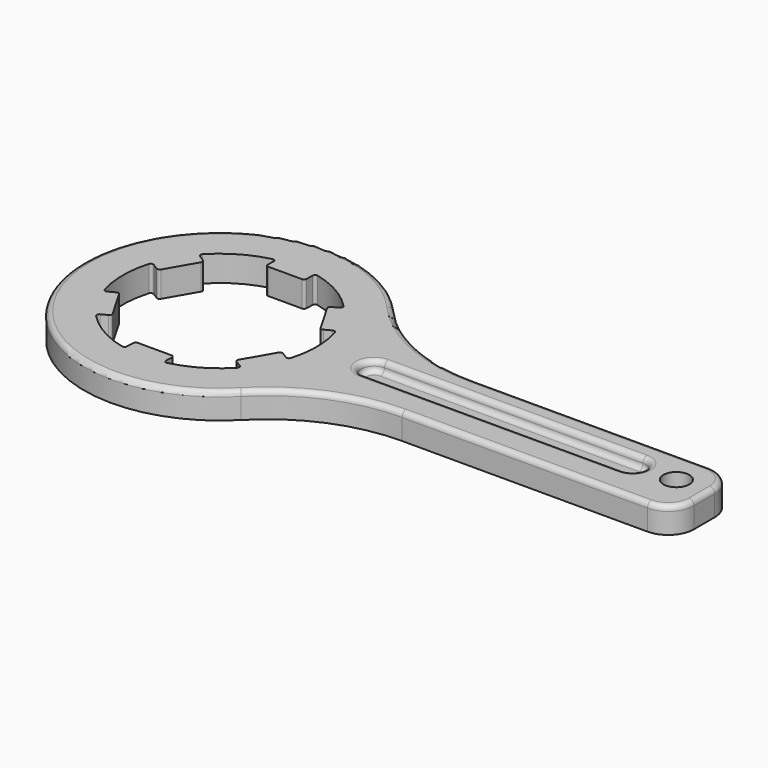
from build123d import *

# Parameters (mm, degrees)
F0_R     = 5
F1_DEPTH = 10
F2_R     = 10
F3_R     = 1
F4_DEPTH = 6
F5_R     = 1.99999
F6_R     = 2


# Not quite as in the source:
# - a fillet or chamfer is up to 0.001 mm smaller than in the source, because OpenCascade refuses the exact size


with BuildPart() as f1:
    # F0 (on Top) → F1 (new body)
    with BuildSketch(Plane.XY):
        with BuildLine():
            ThreePointArc((87.8922518749, 12.982062427), (61.2373823548, 18.6986926605), (39.2710061569, 34.8430491695))
            ThreePointArc((39.2710061569, 34.8430491695), (-52.4855584858, 1.231320604), (37.5938529252, -36.6463125326))
            ThreePointArc((37.5938529252, -36.6463125326), (58.881501719, -22.1257192654), (84.1386232135, -17.017937573))
            Line((84.1386232135, -17.017937573), (188.9996444946, -17.017937573))
            Line((188.9996444946, -17.017937573), (188.9996444946, 12.982062427))
            Line((188.9996444946, 12.982062427), (87.8922518749, 12.982062427))
        make_face()
        with BuildLine():
            ThreePointArc((-28.0871828778, 24.8467333464), (-18.7727000217, 32.4628361961), (-7.5256854941, 36.7370937588))
            Line((-7.5256854941, 36.7370937588), (-7.6951050263, 31.7399648809))
            Line((-7.6951050263, 31.7399648809), (7.3048913079, 31.7504516883))
            Line((7.3048913079, 31.7504516883), (7.4743108401, 36.7475805661))
            ThreePointArc((7.4743108401, 36.7475805661), (18.7272908139, 32.4890532145), (28.0524137093, 24.8859816982))
            Line((28.0524137093, 24.8859816982), (23.6400633889, 22.5341388781))
            Line((23.6400633889, 22.5341388781), (31.1491433976, 9.5490043996))
            Line((31.1491433976, 9.5490043996), (35.561493718, 11.9008472197))
            ThreePointArc((35.561493718, 11.9008472197), (37.4999908356, 0.0262170183), (35.5780992034, -11.8511120606))
            Line((35.5780992034, -11.8511120606), (31.3351684153, -9.2058260029))
            Line((31.3351684153, -9.2058260029), (23.8442520897, -22.2014472886))
            Line((23.8442520897, -22.2014472886), (28.0871828778, -24.8467333464))
            ThreePointArc((28.0871828778, -24.8467333464), (18.7727000217, -32.4628361961), (7.5256854941, -36.7370937588))
            Line((7.5256854941, -36.7370937588), (7.6951050263, -31.7399648809))
            Line((7.6951050263, -31.7399648809), (-7.3048913079, -31.7504516883))
            Line((-7.3048913079, -31.7504516883), (-7.4743108401, -36.7475805661))
            ThreePointArc((-7.4743108401, -36.7475805661), (-18.7272908139, -32.4890532145), (-28.0524137093, -24.8859816982))
            Line((-28.0524137093, -24.8859816982), (-23.6400633889, -22.5341388781))
            Line((-23.6400633889, -22.5341388781), (-31.1491433976, -9.5490043996))
            Line((-31.1491433976, -9.5490043996), (-35.561493718, -11.9008472197))
            ThreePointArc((-35.561493718, -11.9008472197), (-37.4999908356, -0.0262170183), (-35.5780992034, 11.8511120606))
            Line((-35.5780992034, 11.8511120606), (-31.3351684153, 9.2058260029))
            Line((-31.3351684153, 9.2058260029), (-23.8442520897, 22.2014472886))
            Line((-23.8442520897, 22.2014472886), (-28.0871828778, 24.8467333464))
        make_face(mode=Mode.SUBTRACT)
        with BuildLine():
            Line((159.6448034048, -5), (59.6448034048, -5))
            ThreePointArc((59.6448034048, -5), (54.6448034048, 0), (59.6448034048, 5))
            Line((59.6448034048, 5), (159.6448034048, 5))
            ThreePointArc((159.6448034048, 5), (164.6448034048, 0), (159.6448034048, -5))
        make_face(mode=Mode.SUBTRACT)
        with Locations((176.5601634979, 0)):
            Circle(F0_R, mode=Mode.SUBTRACT)
    extrude(amount=F1_DEPTH)

    # F2
    f2_edges = [f1.edges().sort_by_distance(p)[0] for p in [
        (188.999644, 12.982062, 5),
        (188.999644, -17.017938, 5),
    ]]
    fillet(f2_edges, radius=F2_R)

    # F3
    f3_edges = [f1.edges().sort_by_distance(p)[0] for p in [
        (-7.525685, 36.737094, 5),
        (-7.695105, 31.739965, 5),
        (7.304891, 31.750452, 5),
        (7.474311, 36.747581, 5),
        (23.640063, 22.534139, 5),
        (28.052414, 24.885982, 5),
        (31.149143, 9.549004, 5),
        (35.561494, 11.900847, 5),
        (35.578099, -11.851112, 5),
        (31.335168, -9.205826, 5),
        (23.844252, -22.201447, 5),
        (28.087183, -24.846733, 5),
        (7.525685, -36.737094, 5),
        (7.695105, -31.739965, 5),
        (-7.304891, -31.750452, 5),
        (-7.474311, -36.747581, 5),
        (-28.052414, -24.885982, 5),
        (-23.640063, -22.534139, 5),
        (-31.149143, -9.549004, 5),
        (-35.561494, -11.900847, 5),
        (-35.578099, 11.851112, 5),
        (-31.335168, 9.205826, 5),
        (-23.844252, 22.201447, 5),
        (-28.087183, 24.846733, 5),
    ]]
    fillet(f3_edges, radius=F3_R)

    # F0 (on Top) → F4 (join)
    with BuildSketch(Plane.XY):
        with BuildLine():
            ThreePointArc((59.6448034048, 5), (54.6448034048, 0), (59.6448034048, -5))
            Line((59.6448034048, -5), (159.6448034048, -5))
            ThreePointArc((159.6448034048, -5), (164.6448034048, 0), (159.6448034048, 5))
            Line((159.6448034048, 5), (59.6448034048, 5))
        make_face()
    extrude(amount=F4_DEPTH)

    # F5 (radius 2 in the source; OpenCascade refuses exactly that, so slightly less here)
    f5_edges = [f1.edges().sort_by_distance(p)[0] for p in [
        (109.644803, 5, 6),
        (109.644803, 5, 10),
    ]]
    fillet(f5_edges, radius=F5_R)

    # F6
    f6_edges = [f1.edges().sort_by_distance(p)[0] for p in [
        (-52.485558, 1.231321, 10),
    ]]
    fillet(f6_edges, radius=F6_R)


solid = f1.part
